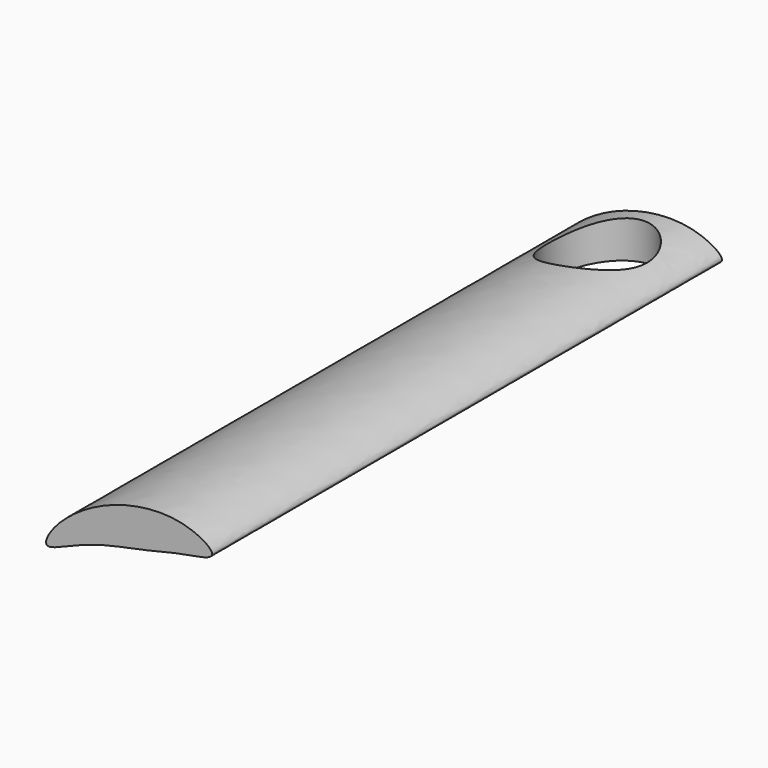
from build123d import *

# Parameters (mm, degrees)
F1_DEPTH = 558.8
F2_R     = 43.6141471532
F3_DEPTH = 76.2


with BuildPart() as f1:
    # F0 (on Front) → F1 (new body)
    with BuildSketch(Plane.XZ):
        with BuildLine():
            add(Edge.make_bspline(
                [(-93.8233584166, 0), (-86.964788528, 10.8961530614), (-53.3488912454, 40.2473774939), (17.1392188212, 53.6933022681), (60.8649370164, 26.727875526), (20.1424094107, 21.802883867), (-9.6864774684, 13.0167223514), (-61.7829224074, 4.4039494215), (-100.6487891792, -16.9596835144), (-96.910600397, -4.9046757126), (-93.8233584166, 0)],
                knots=[0, 0, 0, 0, 0.1491728712, 0.3262065643, 0.4387719772, 0.5407901282, 0.6619668175, 0.8157331914, 0.9328529478, 1, 1, 1, 1], degree=3))
        make_face()
    extrude(amount=F1_DEPTH)

    # F2 (on Top) → F3 (cut)
    with BuildSketch(Plane.XY):
        with Locations((-16.1385573447, -56.0311153531)):
            Circle(F2_R)
    extrude(amount=F3_DEPTH, mode=Mode.SUBTRACT)


solid = f1.part
